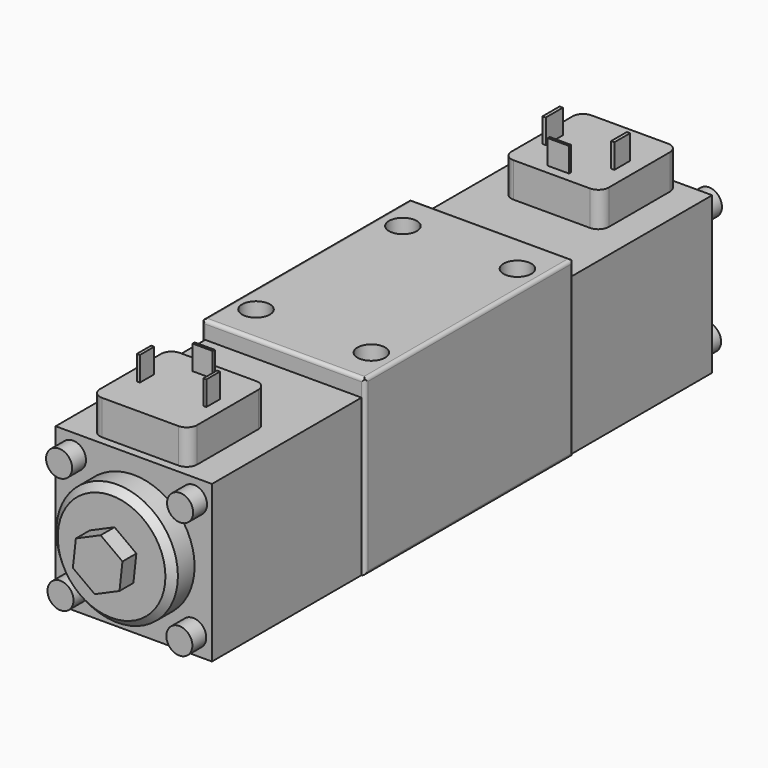
from build123d import *

# Parameters (mm, degrees)
F0_W         = 45
F0_H         = 45
F1_DEPTH     = 180
F2_R         = 17.5
F3_DEPTH     = 8
F4_R         = 17.5
F5_DEPTH     = 8
F7_R         = 3.75
F7_R_2       = 3.7499984493
F8_DEPTH     = 5
F10_DEPTH    = 5
F12_DEPTH    = 5
F13_R        = 3.75
F14_DEPTH    = 5
F15_SIZE     = 2
F16_SIZE     = 2
F18_DEPTH    = 10
F19_W        = 47
F19_H        = 75
F20_DEPTH    = 5
F21_W        = 75
F21_H        = 45
F22_DEPTH    = 1
F23_W        = 75
F23_H        = 45
F24_DEPTH    = 1
F26_R        = 1
F27_T1_DEPTH = 54
F27_T3_DEPTH = 80
F28_T1_DEPTH = 54
F28_T3_DEPTH = 80
F30_W        = 5.8096207213
F30_H        = 0.7481295615
F30_W_2      = 0.8483259007
F30_H_2      = 4.9202227965
F30_W_3      = 0.8840924129
F30_H_3      = 5.1502166316
F31_DEPTH    = 7
F32_W        = 6.1297102366
F32_H        = 0.7072687149
F32_W_2      = 0.9430320933
F32_H_2      = 6.1297118664
F32_W_3      = 0.943031162
F32_H_3      = 5.6581944227
F33_DEPTH    = 7
F34_R        = 3
F35_DEPTH    = 50.0010001
F36_R        = 4
F37_DEPTH    = 6
F38_R        = 3
F39_DEPTH    = 15
F40_R        = 5
F41_DEPTH    = 5


# Not quite as in the source:
# - a fillet or chamfer that OpenCascade refuses, or shapes differently, is made with other operations: its cross-section is extruded or revolved along the edge and cut away or added


with BuildPart() as f1:
    # F0 (on Front) → F1 (new body)
    with BuildSketch(Plane.XZ):
        Rectangle(F0_W, F0_H)
    extrude(amount=-F1_DEPTH)

    # F2 (on face) → F3 (join)
    with BuildSketch(Plane.XZ):
        Circle(F2_R)
    extrude(amount=F3_DEPTH)

    # F4 (on face) → F5 (join)
    with BuildSketch(Plane(origin=(0, 180, 0), x_dir=(-1, 0, 0), z_dir=(0, 1, 0))):
        Circle(F4_R)
    extrude(amount=F5_DEPTH)

    # F7 (on face) → F8 (join)
    with BuildSketch(Plane.XZ):
        with Locations((17.1096809639, -16.9600257193)):
            Circle(F7_R)
        with Locations((-17.0954318406, -16.6246457586)):
            Circle(F7_R_2)
        with Locations((17.3285728585, 16.8300483143)):
            Circle(F7_R)
        with Locations((-17.5076594155, 16.7479507506)):
            Circle(F7_R)
    extrude(amount=F8_DEPTH)

    # F9 (on face) → F10 (join)
    with BuildSketch(Plane.XZ.offset(8)):
        Polygon((0.8549342432, 7.7471986834), (-6.2818037464, 4.6139941149), (-7.1367379896, -3.1332045685), (-0.8549342432, -7.7471986834), (6.2818037464, -4.6139941149), (7.1367379896, 3.1332045685), align=None)
    extrude(amount=F10_DEPTH)

    # F11 (on face) → F12 (join)
    with BuildSketch(Plane(origin=(0, 188, 0), x_dir=(-1, 0, 0), z_dir=(0, 1, 0))):
        Polygon((-6.75, 3.897114317), (-6.75, -3.897114317), (0, -7.7942286341), (6.75, -3.897114317), (6.75, 3.897114317), (0, 7.7942286341), align=None)
    extrude(amount=F12_DEPTH)

    # F13 (on face) → F14 (join)
    with BuildSketch(Plane(origin=(0, 180, 0), x_dir=(-1, 0, 0), z_dir=(0, 1, 0))):
        with Locations((-17.5592578045, 17.1251863153)):
            Circle(F13_R)
        with Locations((17.3599259119, 17.5177720395)):
            Circle(F13_R)
        with Locations((-17.3171540609, -17.1238681393)):
            Circle(F13_R)
        with Locations((17.3687300018, -17.4198415596)):
            Circle(F13_R)
    extrude(amount=F14_DEPTH)

    # F15
    f15_edges = [f1.edges().sort_by_distance(p)[0] for p in [
        (-17.5, -8, 0),
    ]]
    chamfer(f15_edges, length=F15_SIZE)

    # F16
    f16_edges = [f1.edges().sort_by_distance(p)[0] for p in [
        (17.5, 188, 0),
    ]]
    chamfer(f16_edges, length=F16_SIZE)

    # F17 (on face) → F18 (join)
    with BuildSketch(Plane.XY.offset(22.5)):
        with BuildLine():
            Line((-11, 150.4180943225), (11, 150.4180943225))
            ThreePointArc((11, 150.4180943225), (13.1213203436, 151.296773979), (14, 153.4180943225))
            Line((14, 153.4180943225), (14, 175.4180943225))
            ThreePointArc((14, 175.4180943225), (13.1213203436, 177.5394146661), (11, 178.4180943225))
            Line((11, 178.4180943225), (-11, 178.4180943225))
            ThreePointArc((-11, 178.4180943225), (-13.1213203436, 177.5394146661), (-14, 175.4180943225))
            Line((-14, 175.4180943225), (-14, 153.4180943225))
            ThreePointArc((-14, 153.4180943225), (-13.1213203436, 151.296773979), (-11, 150.4180943225))
        make_face()
        with BuildLine():
            Line((11, 30.3079142428), (-11, 30.3079142428))
            ThreePointArc((-11, 30.3079142428), (-13.1213203436, 29.4292345863), (-14, 27.3079142428))
            Line((-14, 27.3079142428), (-14, 5.3079142428))
            ThreePointArc((-14, 5.3079142428), (-13.1213203436, 3.1865938992), (-11, 2.3079142428))
            Line((-11, 2.3079142428), (11, 2.3079142428))
            ThreePointArc((11, 2.3079142428), (13.1213203436, 3.1865938992), (14, 5.3079142428))
            Line((14, 5.3079142428), (14, 27.3079142428))
            ThreePointArc((14, 27.3079142428), (13.1213203436, 29.4292345863), (11, 30.3079142428))
        make_face()
    extrude(amount=F18_DEPTH)

    # F19 (on face) → F20 (join)
    with BuildSketch(Plane.XY.offset(22.5)):
        with Locations((0, 91.3310141564)):
            Rectangle(F19_W, F19_H)
    extrude(amount=F20_DEPTH)

    # F21 (on face) → F22 (join)
    with BuildSketch(Plane.YZ.offset(22.5)):
        with Locations((91.3310141564, 0)):
            Rectangle(F21_W, F21_H)
    extrude(amount=F22_DEPTH)

    # F23 (on face) → F24 (join)
    with BuildSketch(Plane(origin=(-22.5, 0, 0), x_dir=(0, -1, 0), z_dir=(-1, 0, 0))):
        with Locations((-91.3310141564, 0)):
            Rectangle(F23_W, F23_H)
    extrude(amount=F24_DEPTH)

    # F26
    f26_edges = [f1.edges().sort_by_distance(p)[0] for p in [
        (23.5, 91.331014, 27.5),
        (0, 128.831014, 27.5),
        (-23.5, 91.331014, 27.5),
        (0, 53.831014, 27.5),
    ]]
    fillet(f26_edges, radius=F26_R)

    # F27: fillet of radius 1 on 4 edges, made by hand

    # F27_s2 → F27_t1 (cut)
    with BuildSketch(Plane.XY.offset(-25)):
        with BuildLine():
            ThreePointArc((-22.5, 53.8310141564), (-23.2071067812, 54.1239073753), (-23.5, 54.8310141564))
            Line((-23.5, 54.8310141564), (-23.5, 53.8310141564))
            Line((-23.5, 53.8310141564), (-22.5, 53.8310141564))
        make_face()
        with BuildLine():
            ThreePointArc((-22.5, 128.8310141564), (-23.2071067812, 128.5381209376), (-23.5, 127.8310141564))
            Line((-23.5, 127.8310141564), (-23.5, 128.8310141564))
            Line((-23.5, 128.8310141564), (-22.5, 128.8310141564))
        make_face()
    extrude(amount=F27_T1_DEPTH, mode=Mode.SUBTRACT)

    # F27_s4 → F27_t3 (cut)
    with BuildSketch(Plane.XZ.offset(-131.3310141564)):
        with BuildLine():
            ThreePointArc((-22.5, -22.5), (-23.2071067812, -22.2071067812), (-23.5, -21.5))
            Line((-23.5, -21.5), (-23.5, -22.5))
            Line((-23.5, -22.5), (-22.5, -22.5))
        make_face()
    extrude(amount=F27_T3_DEPTH, mode=Mode.SUBTRACT)

    # F28: fillet of radius 1 on 4 edges, made by hand

    # F28_s2 → F28_t1 (cut)
    with BuildSketch(Plane.XY.offset(-25)):
        with BuildLine():
            ThreePointArc((23.5, 54.8310141564), (23.2071067812, 54.1239073753), (22.5, 53.8310141564))
            Line((22.5, 53.8310141564), (23.5, 53.8310141564))
            Line((23.5, 53.8310141564), (23.5, 54.8310141564))
        make_face()
        with BuildLine():
            ThreePointArc((23.5, 127.8310141564), (23.2071067812, 128.5381209376), (22.5, 128.8310141564))
            Line((22.5, 128.8310141564), (23.5, 128.8310141564))
            Line((23.5, 128.8310141564), (23.5, 127.8310141564))
        make_face()
    extrude(amount=F28_T1_DEPTH, mode=Mode.SUBTRACT)

    # F28_s4 → F28_t3 (cut)
    with BuildSketch(Plane.XZ.offset(-131.3310141564)):
        with BuildLine():
            ThreePointArc((23.5, -21.5), (23.2071067812, -22.2071067812), (22.5, -22.5))
            Line((22.5, -22.5), (23.5, -22.5))
            Line((23.5, -22.5), (23.5, -21.5))
        make_face()
    extrude(amount=F28_T3_DEPTH, mode=Mode.SUBTRACT)

    # F30 (on face) → F31 (join)
    with BuildSketch(Plane.XY.offset(32.5)):
        with Locations((-0.3073244588, 25.5132811144)):
            Rectangle(F30_W, F30_H)
        with Locations((9.7066606395, 15.8806457184)):
            Rectangle(F30_W_2, F30_H_2)
        with Locations((-9.4111547805, 15.995642636)):
            Rectangle(F30_W_3, F30_H_3)
    extrude(amount=F31_DEPTH)

    # F32 (on face) → F33 (join)
    with BuildSketch(Plane.XY.offset(32.5)):
        with Locations((-0.2737542382, 153.4767895937)):
            Rectangle(F32_W, F32_H)
        with Locations((-10.4113533162, 163.7322604656)):
            Rectangle(F32_W_2, F32_H_2)
        with Locations((9.1565707698, 163.7322679162)):
            Rectangle(F32_W_3, F32_H_3)
    extrude(amount=F33_DEPTH)

    # F34 (on face) → F35 (cut, through all)
    with BuildSketch(Plane.XY.offset(27.5)):
        with Locations((-16.4304438433, 117.3707548044)):
            Circle(F34_R)
        with Locations((16.6706163436, 117.2029972076)):
            Circle(F34_R)
        with Locations((-16.8373230845, 65.0239661336)):
            Circle(F34_R)
        with Locations((16.5224820375, 64.8282542825)):
            Circle(F34_R)
    extrude(amount=-F35_DEPTH, mode=Mode.SUBTRACT)

    # F36 (on face) → F37 (cut)
    with BuildSketch(Plane.XY.offset(27.5)):
        with Locations((-16.4304438433, 117.3707548044)):
            Circle(F36_R)
        with Locations((16.6706163436, 117.2029972076)):
            Circle(F36_R)
        with Locations((-16.8373230845, 65.0239661336)):
            Circle(F36_R)
        with Locations((16.5224820375, 64.8282542825)):
            Circle(F36_R)
    extrude(amount=-F37_DEPTH, mode=Mode.SUBTRACT)

    # F38 (on face) → F39 (cut)
    with BuildSketch(Plane(origin=(0, 0, -22.5), x_dir=(1, 0, 0), z_dir=(0, 0, -1))):
        with Locations((9.9463667721, -91.3435295224)):
            Circle(F38_R)
        with Locations((0, -83.0129310489)):
            Circle(F38_R)
        with Locations((-9.6791982651, -91.0631641746)):
            Circle(F38_R)
        with Locations((0, -99.4741246104)):
            Circle(F38_R)
    extrude(amount=-F39_DEPTH, mode=Mode.SUBTRACT)

    # F40 (on face) → F41 (cut)
    with BuildSketch(Plane(origin=(0, 0, -22.5), x_dir=(1, 0, 0), z_dir=(0, 0, -1))):
        with Locations((-9.6358787246, -91.2054658611)):
            Circle(F40_R)
        with Locations((0, -83.0830261111)):
            Circle(F40_R)
        with Locations((9.9296290427, -91.4075896144)):
            Circle(F40_R)
        with Locations((0, -99.3979945779)):
            Circle(F40_R)
    extrude(amount=-F41_DEPTH, mode=Mode.SUBTRACT)


solid = f1.part
